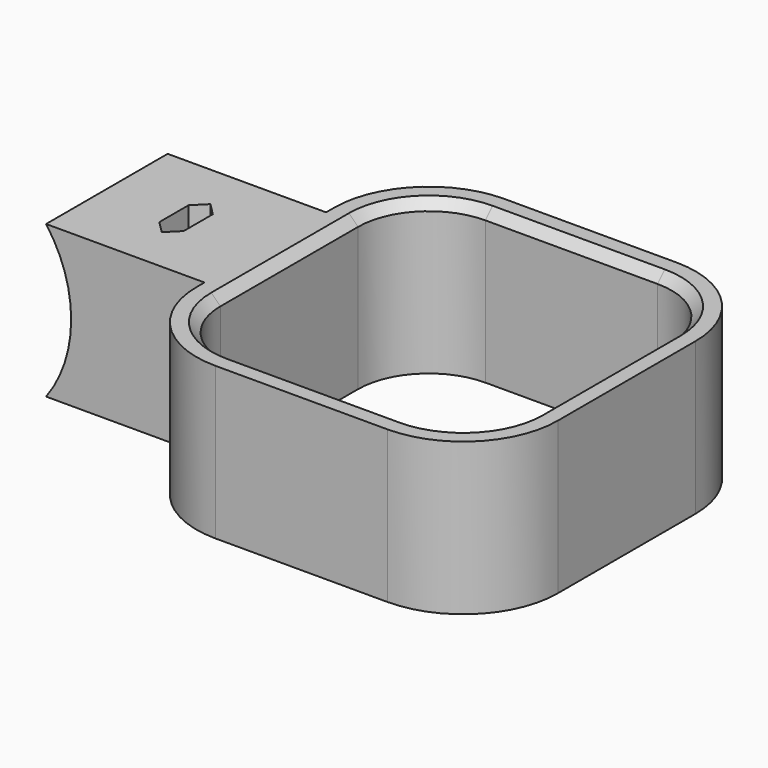
from build123d import *

# Parameters (mm, degrees)
F0_W     = 2
F0_H     = 12.7
F0_W_2   = 13.24
F1_DEPTH = 12.7
F3_DEPTH = 12.7
F4_W     = 2.032
F4_H     = 5.08
F5_DEPTH = 12.7
F6_SIZE  = 1.01599
F7_SIZE  = 0.762


# Not quite as in the source:
# - a fillet or chamfer is up to 0.001 mm smaller than in the source, because OpenCascade refuses the exact size


with BuildPart() as f1:
    # F0 (on Top) → F1 (new body)
    with BuildSketch(Plane.XY):
        with Locations((-14.1, 0)):
            Rectangle(F0_W, F0_H)
        with Locations((-21.72, 0)):
            Rectangle(F0_W_2, F0_H)
        with BuildLine():
            ThreePointArc((7.19, 13.1), (11.3690010768, 11.3690010768), (13.1, 7.19))
            Line((13.1, 7.19), (13.1, -7.19))
            ThreePointArc((13.1, -7.19), (11.3690010768, -11.3690010768), (7.19, -13.1))
            Line((7.19, -13.1), (-7.19, -13.1))
            ThreePointArc((-7.19, -13.1), (-11.3690010768, -11.3690010768), (-13.1, -7.19))
            Line((-13.1, -7.19), (-13.1, -6.35))
            Line((-13.1, -6.35), (-15.1, -6.35))
            Line((-15.1, -6.35), (-15.1, -7.19))
            ThreePointArc((-15.1, -7.19), (-12.7832146392, -12.7832146392), (-7.19, -15.1))
            Line((-7.19, -15.1), (7.19, -15.1))
            ThreePointArc((7.19, -15.1), (12.7832146392, -12.7832146392), (15.1, -7.19))
            Line((15.1, -7.19), (15.1, 7.19))
            ThreePointArc((15.1, 7.19), (12.7832146392, 12.7832146392), (7.19, 15.1))
            Line((7.19, 15.1), (-7.19, 15.1))
            ThreePointArc((-7.19, 15.1), (-12.7832146392, 12.7832146392), (-15.1, 7.19))
            Line((-15.1, 7.19), (-15.1, 6.35))
            Line((-15.1, 6.35), (-13.1, 6.35))
            Line((-13.1, 6.35), (-13.1, 7.19))
            ThreePointArc((-13.1, 7.19), (-11.3690010768, 11.3690010768), (-7.19, 13.1))
            Line((-7.19, 13.1), (7.19, 13.1))
        make_face()
    extrude(amount=F1_DEPTH)

    # F2 (on face) → F3 (cut, through all)
    with BuildSketch(Plane.XZ.offset(6.35)):
        with BuildLine():
            ThreePointArc((-28.34, 0), (-26.7817380481, 3.0065509582), (-26.2442648116, 6.35))
            ThreePointArc((-26.2442648116, 6.35), (-26.7817380481, 9.6934490418), (-28.34, 12.7))
            Line((-28.34, 12.7), (-28.34, 0))
        make_face()
    extrude(amount=-F3_DEPTH, mode=Mode.SUBTRACT)

    # F4 (on face) → F5 (cut, through all)
    with BuildSketch(Plane.XY.offset(12.7)):
        with Locations((-21.72, 0)):
            Rectangle(F4_W, F4_H)
    extrude(amount=-F5_DEPTH, mode=Mode.SUBTRACT)

    # F6 (size 1.016 in the source; OpenCascade refuses exactly that, so slightly less here)
    f6_edges = [f1.edges().sort_by_distance(p)[0] for p in [
        (-22.736, -2.54, 6.35),
        (-20.704, -2.54, 6.35),
        (-20.704, 2.54, 6.35),
        (-22.736, 2.54, 6.35),
    ]]
    chamfer(f6_edges, length=F6_SIZE)

    # F7
    f7_edges = [f1.edges().sort_by_distance(p)[0] for p in [
        (-11.369001, -11.369001, 12.7),
        (0, -13.1, 12.7),
        (-13.1, 0, 12.7),
        (-11.369001, 11.369001, 12.7),
        (0, 13.1, 12.7),
        (11.369001, 11.369001, 12.7),
        (13.1, 0, 12.7),
        (11.369001, -11.369001, 12.7),
    ]]
    chamfer(f7_edges, length=F7_SIZE)


solid = f1.part
